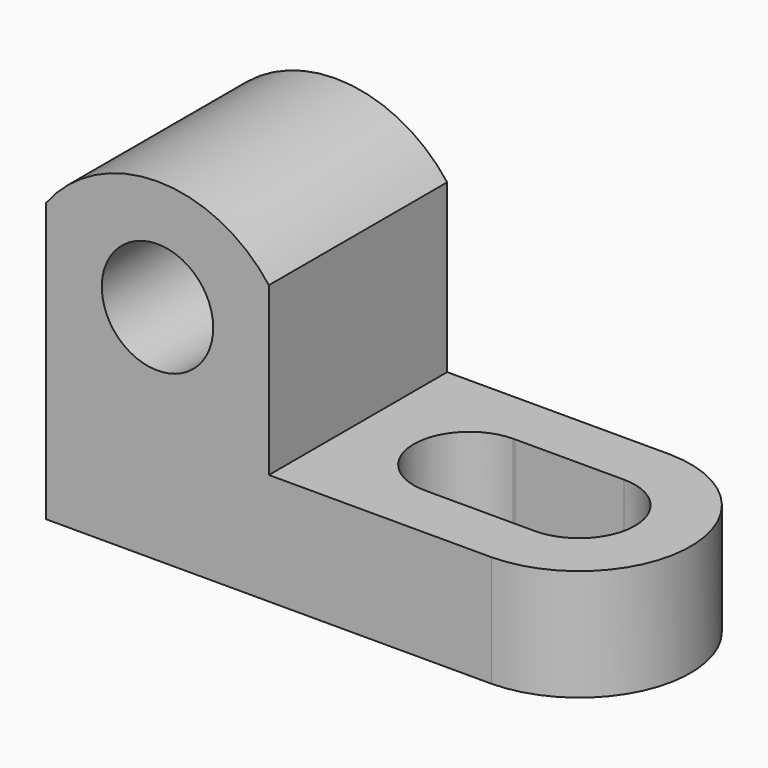
from build123d import *

# Parameters (mm, degrees)
F1_DEPTH = 25.4
F2_R     = 6.35
F3_DEPTH = 25.4
F5_DEPTH = 25.4
F7_DEPTH = 25.4


with BuildPart() as f1:
    # F0 (on Front) → F1 (new body)
    with BuildSketch(Plane.XZ):
        Polygon((0, 38.1), (0, 0), (63.5, 0), (63.5, 12.7), (25.4, 12.7), (25.4, 38.1), align=None)
    extrude(amount=F1_DEPTH)

    # F2 (on face) → F3 (cut)
    with BuildSketch(Plane.XZ.offset(25.4)):
        with BuildLine():
            Line((0, 38.1), (0, 31.75))
            ThreePointArc((0, 31.75), (12.7, 38.0364069073), (25.4, 31.75))
            Line((25.4, 31.75), (25.4, 38.1))
            Line((25.4, 38.1), (0, 38.1))
        make_face()
        with Locations((12.7, 25.4)):
            Circle(F2_R)
    extrude(amount=-F3_DEPTH, mode=Mode.SUBTRACT)

    # F4 (on face) → F5 (cut)
    with BuildSketch(Plane.XY.offset(12.7)):
        with BuildLine():
            ThreePointArc((50.8, 0), (63.3139332649, -12.7), (50.8, -25.4))
            Line((50.8, -25.4), (63.5, -25.4))
            Line((63.5, -25.4), (63.5, 0))
            Line((63.5, 0), (50.8, 0))
        make_face()
    extrude(amount=-F5_DEPTH, mode=Mode.SUBTRACT)

    # F6 (on face) → F7 (cut)
    with BuildSketch(Plane.XY.offset(12.7)):
        with BuildLine():
            Line((38.236319864, -6.3514592475), (37.9621789193, -6.3514916602))
            ThreePointArc((37.9621789193, -6.3514916602), (31.7513794229, -12.8323467712), (38.2268806789, -19.048728101))
            ThreePointArc((38.2268806789, -19.048728101), (42.2376787534, -17.5168531718), (44.3569666293, -13.7829864238))
            ThreePointArc((44.3569666293, -13.7829864238), (44.2639332586, -12.6999958422), (44.3569666293, -11.6170052607))
            ThreePointArc((44.3569666293, -11.6170052607), (42.2412584743, -7.8862158048), (38.236319864, -6.3514592475))
        make_face()
        with BuildLine():
            ThreePointArc((44.3569666293, -13.7829864238), (42.2376787534, -17.5168531718), (38.2268806789, -19.048728101))
            Line((38.2268806789, -19.048728101), (50.6132833568, -19.049995809))
            ThreePointArc((50.6132833568, -19.049995809), (46.5243381529, -17.5577434552), (44.3569666293, -13.7829864238))
        make_face()
        with BuildLine():
            Line((50.6131824753, -6.3499958866), (38.236319864, -6.3514592475))
            ThreePointArc((38.236319864, -6.3514592475), (42.2412584743, -7.8862158048), (44.3569666293, -11.6170052607))
            ThreePointArc((44.3569666293, -11.6170052607), (46.5242995659, -7.8422807148), (50.6131824753, -6.3499958866))
        make_face()
        with BuildLine():
            ThreePointArc((44.3569666293, -11.6170052607), (44.2639332586, -12.6999958422), (44.3569666293, -13.7829864238))
            ThreePointArc((44.3569666293, -13.7829864238), (44.4266989061, -13.2434854483), (44.45, -12.6999958422))
            ThreePointArc((44.45, -12.6999958422), (44.4266989061, -12.1565062361), (44.3569666293, -11.6170052607))
        make_face()
        with BuildLine():
            ThreePointArc((44.45, -12.6999958422), (44.4266989061, -13.2434854483), (44.3569666293, -13.7829864238))
            ThreePointArc((44.3569666293, -13.7829864238), (46.5243381529, -17.5577434552), (50.6132833568, -19.049995809))
            ThreePointArc((50.6132833568, -19.049995809), (55.1038315383, -17.1903536719), (56.9639332586, -12.6999958422))
            ThreePointArc((56.9639332586, -12.6999958422), (55.1037958693, -8.2096023476), (50.6131824753, -6.3499958866))
            ThreePointArc((50.6131824753, -6.3499958866), (46.5242995659, -7.8422807148), (44.3569666293, -11.6170052607))
            ThreePointArc((44.3569666293, -11.6170052607), (44.4266989061, -12.1565062361), (44.45, -12.6999958422))
        make_face()
    extrude(amount=-F7_DEPTH, mode=Mode.SUBTRACT)


solid = f1.part
